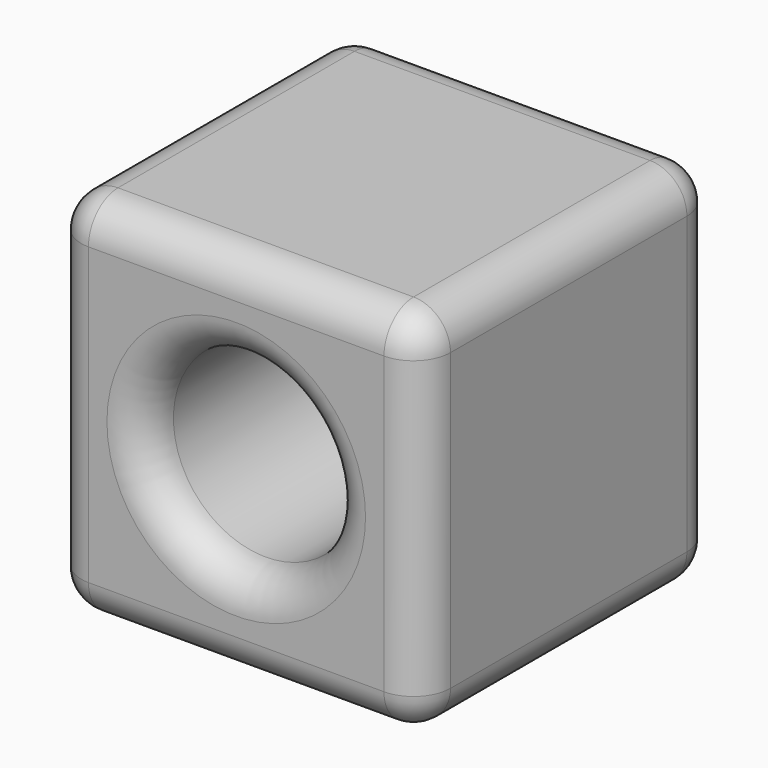
from build123d import *

# Parameters (mm, degrees)
F0_W     = 50
F0_H     = 50
F1_DEPTH = 50
F2_R     = 12.5
F3_DEPTH = 50.001
F4_R     = 5
F5_R     = 5


with BuildPart() as f1:
    # F0 (on Top) → F1 (new body)
    with BuildSketch(Plane.XY):
        Rectangle(F0_W, F0_H)
    extrude(amount=F1_DEPTH)

    # F2 (on face) → F3 (cut, through all)
    with BuildSketch(Plane.XZ.offset(25)):
        with Locations((0, 25)):
            Circle(F2_R)
    extrude(amount=-F3_DEPTH, mode=Mode.SUBTRACT)

    # F4
    f4_edges = [f1.edges().sort_by_distance(p)[0] for p in [
        (0, -25, 50),
        (-25, 0, 50),
        (0, 25, 50),
        (25, 0, 50),
        (25, 25, 25),
        (25, -25, 25),
        (25, 0, 0),
        (0, -25, 0),
        (-25, -25, 25),
        (-25, 0, 0),
        (0, 25, 0),
        (-25, 25, 25),
    ]]
    fillet(f4_edges, radius=F4_R)

    # F5
    f5_edges = [f1.edges().sort_by_distance(p)[0] for p in [
        (-12.5, -25, 25),
        (25, 0, 5),
        (20, 0, 0),
        (0, 20, 0),
        (-12.5, 25, 25),
    ]]
    fillet(f5_edges, radius=F5_R)


solid = f1.part
